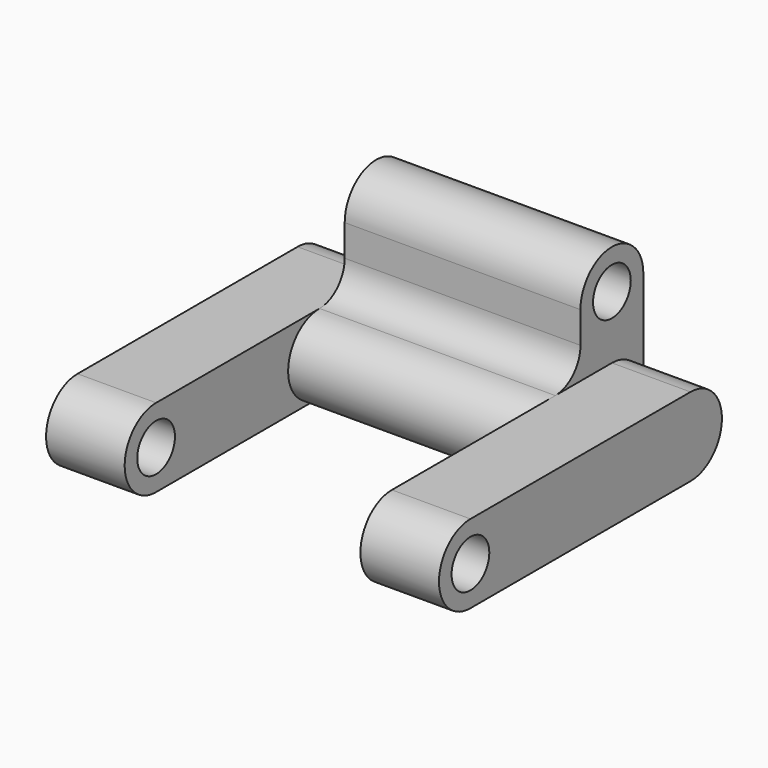
from build123d import *

# Parameters (mm, degrees)
F0_R     = 1.5
F1_DEPTH = 7.5
F2_R     = 1.5
F3_DEPTH = 5
F4_R     = 2.4999


# Not quite as in the source:
# - a fillet or chamfer is up to 0.001 mm smaller than in the source, because OpenCascade refuses the exact size
# - a pattern or mirror of a feature is missing from the dataset's text; its kind, count and spacing are read off the source's solid


with BuildPart() as f1:
    # F0 (on Right) → F1 (new body, symmetric)
    with BuildSketch(Plane.YZ):
        with BuildLine():
            Line((-4.5, -0.685833849), (-2.5, -0.685833849))
            Line((-2.5, -0.685833849), (2.5, -0.685833849))
            Line((2.5, -0.685833849), (2.5, 8.314166151))
            ThreePointArc((2.5, 8.314166151), (0, 10.814166151), (-2.5, 8.314166151))
            Line((-2.5, 8.314166151), (-2.5, 6.314166151))
            ThreePointArc((-2.5, 6.314166151), (-3.0857864376, 4.8999525886), (-4.5, 4.314166151))
            ThreePointArc((-4.5, 4.314166151), (-7, 1.814166151), (-4.5, -0.685833849))
        make_face()
        with Locations((0, 8.314166151)):
            Circle(F0_R, mode=Mode.SUBTRACT)
    extrude(amount=F1_DEPTH, both=True)

    # F2 (on face) → F3 (join)
    with BuildSketch(Plane.YZ.offset(7.5)):
        with BuildLine():
            Line((-17.5, -0.685833849), (0, -0.685833849))
            ThreePointArc((0, -0.685833849), (2.5, 1.814166151), (0, 4.314166151))
            Line((0, 4.314166151), (-17.5, 4.314166151))
            ThreePointArc((-17.5, 4.314166151), (-20, 1.814166151), (-17.5, -0.685833849))
        make_face()
        with Locations((-17.5, 1.814166151)):
            Circle(F2_R, mode=Mode.SUBTRACT)
    f3 = extrude(amount=F3_DEPTH)

    # F3_copies: F3 across plane
    add(f3.mirror(Plane(origin=(0, 0, 0), x_dir=(0, 0, -1), z_dir=(-1, 0, 0))))

    # F4 (radius 2.5 in the source; OpenCascade refuses exactly that, so slightly less here)
    f4_edges = [f1.edges().sort_by_distance(p)[0] for p in [
        (0, 2.5, -0.685834),
    ]]
    fillet(f4_edges, radius=F4_R)


solid = f1.part
